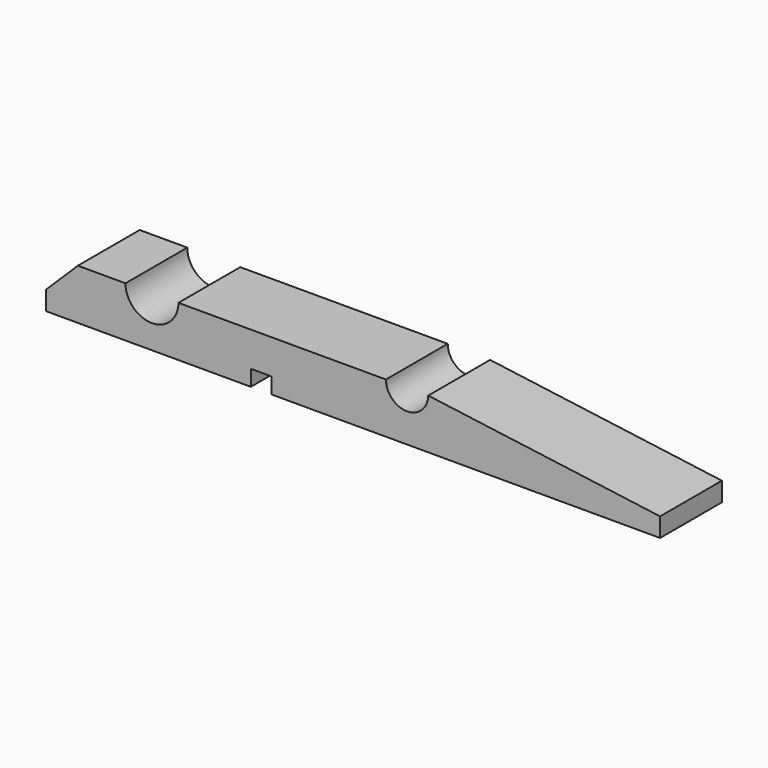
from build123d import *

# Parameters (mm, degrees)
F1_DEPTH     = 9.271
F2_TEXT_SIZE = 5.8208333333
F3_DEPTH     = 0.635


# Not quite as in the source:
# - Text() gives the source's letters only with a copy of the font that has no kerning and outlines rounded to 1/6400 em; it was checked with that copy


with BuildPart() as f1:
    # F0 (on Front) → F1 (new body)
    with BuildSketch(Plane.XZ):
        with BuildLine():
            Line((-10.8983474945, 0), (-10.8983474945, -2.286))
            Line((-10.8983474945, -2.286), (13.6634525055, -2.286))
            Line((13.6634525055, -2.286), (13.6634525055, -0.381))
            Line((13.6634525055, -0.381), (16.1526525055, -0.381))
            Line((16.1526525055, -0.381), (16.1526525055, -2.286))
            Line((16.1526525055, -2.286), (62.7616525055, -2.286))
            Line((62.7616525055, -2.286), (62.7616525055, 0))
            Line((62.7616525055, 0), (34.9482102462, 3.7118029345))
            ThreePointArc((34.9482102462, 3.7118029345), (32.3849529411, 1.2193105672), (29.8686525055, 3.7592))
            Line((29.8686525055, 3.7592), (4.9766525055, 3.7592))
            ThreePointArc((4.9766525055, 3.7592), (1.8016525055, 0.5842), (-1.3733474945, 3.7592))
            Line((-1.3733474945, 3.7592), (-7.0883474945, 3.7592))
            Line((-7.0883474945, 3.7592), (-10.8983474945, 0))
        make_face()
    extrude(amount=F1_DEPTH)

    # F2 (on face) → F3 (cut)
    with BuildSketch(Plane(origin=(0, 0, -2.286), x_dir=(1, 0, 0), z_dir=(0, 0, -1))):
        with Locations((28.8526525055, 2.54)):
            Text('Burghy', F2_TEXT_SIZE, font='Open Sans', font_style=FontStyle.BOLD, text_align=(TextAlign.LEFT, TextAlign.BOTTOM))
    extrude(amount=-F3_DEPTH, mode=Mode.SUBTRACT)


solid = f1.part
